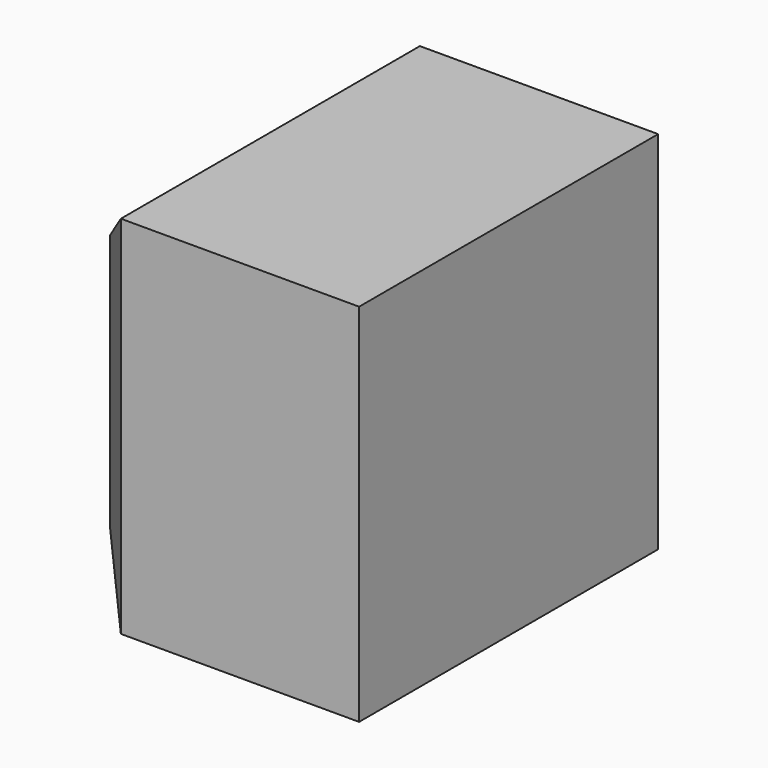
from build123d import *

# Parameters (mm, degrees)
F1_E0_BOTTOM_W = 27.100160718
F1_E0_BOTTOM_H = 34.544
F2_DEPTH       = 33.782
F3_SIZE        = 5.08


with BuildPart() as f2:
    # F1_E0_bottom (on explicit) → F2 (new body)
    with BuildSketch(Plane(origin=(-50.1445159316, 0, -21.0164524615), x_dir=(1, 0, 0), z_dir=(0, 0, -1))):
        with Locations((13.550080359, 17.272)):
            Rectangle(F1_E0_BOTTOM_W, F1_E0_BOTTOM_H)
    extrude(amount=F2_DEPTH)

    # F3
    f3_edges = [f2.edges().sort_by_distance(p)[0] for p in [
        (-50.144516, -34.544, -37.907452),
        (-50.144516, 0, -37.907452),
        (-50.144516, -17.272, -21.016452),
        (-50.144516, -17.272, -54.798452),
    ]]
    chamfer(f3_edges, length=F3_SIZE)


solid = f2.part
